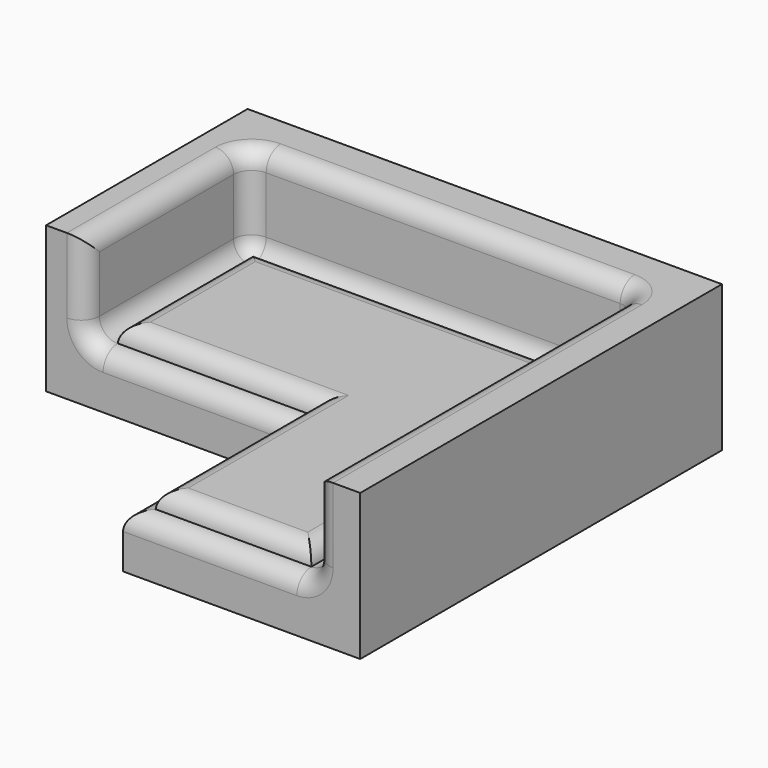
from build123d import *

# Parameters (mm, degrees)
F0_W          = 132.9678967595
F0_H          = 40.9901021048
F1_DEPTH      = 35.306
F2_W          = 109.3940883875
F2_H          = 52.1104875952
F3_DEPTH      = 57.15
F4_W          = 66.4839483798
F4_H          = 40.9901021048
F5_DEPTH      = 56.134
F6_W          = 53.8083352149
F6_H          = 26.0552437976
F7_DEPTH      = 59.69
F8_F1_R       = 5.08
F8_F2_R       = 5.08
F9_W          = 99.2340883875
F9_H          = 46.9125229284
F10_DEPTH     = 4.826
F11_W         = 43.6483352149
F11_H         = 56.2114770716
F12_DEPTH     = 4.826
F13_T1_DEPTH  = 56.3324502806
F13_T3_DEPTH  = 0.0774771487
F13_T5_DEPTH  = 68.8181149887
F13_T7_DEPTH  = 55.5857531726
F13_T9_DEPTH  = 115.8081150657
F13_T11_DEPTH = 99.2340883875
F13_T13_DEPTH = 59.5966379941
F13_T19_DEPTH = 68.2698682383
F13_T23_DEPTH = 12.7615922144


# Not quite as in the source:
# - a fillet or chamfer that OpenCascade refuses, or shapes differently, is made with other operations: its cross-section is extruded or revolved along the edge and cut away or added


with BuildPart() as f1:
    # F0 (on Front) → F1 (new body, symmetric)
    with BuildSketch(Plane.XZ):
        with Locations((0.8887089789, -5.8075287379)):
            Rectangle(F0_W, F0_H)
    extrude(amount=F1_DEPTH, both=True)

    # F2 (on face) → F3 (cut)
    with BuildSketch(Plane.XZ.offset(35.306)):
        with Locations((0, 14.6875223145)):
            Rectangle(F2_W, F2_H)
    extrude(amount=-F3_DEPTH, mode=Mode.SUBTRACT)

    # F4 (on face) → F5 (join)
    with BuildSketch(Plane.XZ.offset(35.306)):
        with Locations((34.1306831688, -5.8075287379)):
            Rectangle(F4_W, F4_H)
    extrude(amount=F5_DEPTH)

    # F6 (on face) → F7 (cut)
    with BuildSketch(Plane(origin=(0, -35.306, 0), x_dir=(-1, 0, 0), z_dir=(0, 1, 0))):
        with Locations((-27.7928765863, 1.6599004157)):
            Rectangle(F6_W, F6_H)
    extrude(amount=-F7_DEPTH, mode=Mode.SUBTRACT)

    # F8: fillet of radius 5.08 on 11 edges, made by hand

    # F8_f1
    f8_f1_edges = [f1.edges().sort_by_distance(p)[0] for p in [
        (-54.6970441937, -6.731, -11.3677214831),
        (-54.6970441937, 21.844, 1.6599004157),
        (0, 21.844, -11.3677214831),
        (54.6970441937, -34.798, -11.3677214831),
        (54.6970441937, 21.844, 1.6599004157),
    ]]
    fillet(f8_f1_edges, radius=F8_F1_R)

    # F8_f2
    f8_f2_edges = [f1.edges().sort_by_distance(p)[0] for p in [
        (-54.6970441937, -9.271, 14.6875223145),
        (0, 21.844, 14.6875223145),
        (54.6970441937, -37.338, 14.6875223145),
        (-24.3641676074, -35.306, -11.3677214831),
        (0.8887089789, -63.373, -11.3677214831),
        (25.2528765863, -91.44, -11.3677214831),
        (53.2091466422, -91.44, -9.8798239315),
        (-53.2091466422, -35.306, -9.8798239315),
        (53.2091466422, 20.3561024484, 14.6875223145),
        (-53.2091466422, 20.3561024484, 14.6875223145),
    ]]
    fillet(f8_f2_edges, radius=F8_F2_R)

    # F9 (on face) → F10 (join)
    with BuildSketch(Plane.XY.offset(-11.3677214831)):
        with Locations((0, -6.6922614642)):
            Rectangle(F9_W, F9_H)
    extrude(amount=F10_DEPTH)

    # F11 (on face) → F12 (join)
    with BuildSketch(Plane.XY.offset(-11.3677214831)):
        with Locations((27.7928765863, -58.2542614642)):
            Rectangle(F11_W, F11_H)
    extrude(amount=F12_DEPTH)

    # F13: fillet of radius 5.08 on 6 edges, made by hand

    # F13_s2 → F13_t1 (cut)
    with BuildSketch(Plane.YZ.offset(-6.7154060868)):
        with BuildLine():
            ThreePointArc((-81.2863539737, -6.5417214831), (-84.7875023567, -7.9409117896), (-86.36, -11.3677214831))
            Line((-86.36, -11.3677214831), (-86.36, -6.5417214831))
            Line((-86.36, -6.5417214831), (-81.2863539737, -6.5417214831))
        make_face()
    extrude(amount=F13_T1_DEPTH, mode=Mode.SUBTRACT)

    # F13_s4 → F13_t3 (cut)
    with BuildSketch(Plane.XZ.offset(30.1485229284)):
        with BuildLine():
            ThreePointArc((11.0423550052, -6.5417214831), (7.5412066221, -7.9409117896), (5.9687089789, -11.3677214831))
            Line((5.9687089789, -11.3677214831), (5.9687089789, -6.5417214831))
            Line((5.9687089789, -6.5417214831), (11.0423550052, -6.5417214831))
        make_face()
    extrude(amount=F13_T3_DEPTH, mode=Mode.SUBTRACT)

    # F13_s6 → F13_t5 (cut)
    with BuildSketch(Plane.XZ.offset(30.226000077)):
        with BuildLine():
            ThreePointArc((11.0423550052, -6.5417214831), (7.5412066221, -7.9409117896), (5.9687089789, -11.3677214831))
            Line((5.9687089789, -11.3677214831), (5.9687089789, -6.5417214831))
            Line((5.9687089789, -6.5417214831), (11.0423550052, -6.5417214831))
        make_face()
    extrude(amount=F13_T5_DEPTH, mode=Mode.SUBTRACT)

    # F13_s8 → F13_t7 (cut)
    with BuildSketch(Plane.YZ.offset(-49.6170441937)):
        with BuildLine():
            ThreePointArc((-25.0748769021, -6.5417214831), (-28.5760252851, -7.9409117896), (-30.1485229284, -11.3677214831))
            Line((-30.1485229284, -11.3677214831), (-30.1485229284, -6.5417214831))
            Line((-30.1485229284, -6.5417214831), (-25.0748769021, -6.5417214831))
        make_face()
    extrude(amount=F13_T7_DEPTH, mode=Mode.SUBTRACT)

    # F13_s10 → F13_t9 (cut)
    with BuildSketch(Plane.XZ.offset(-16.764)):
        with BuildLine():
            ThreePointArc((44.5433981675, -6.5417214831), (48.0445465505, -7.9409117896), (49.6170441937, -11.3677214831))
            Line((49.6170441937, -11.3677214831), (49.6170441937, -6.5417214831))
            Line((49.6170441937, -6.5417214831), (44.5433981675, -6.5417214831))
        make_face()
    extrude(amount=F13_T9_DEPTH, mode=Mode.SUBTRACT)

    # F13_s12 → F13_t11 (cut)
    with BuildSketch(Plane.YZ.offset(-49.6170441937)):
        with BuildLine():
            ThreePointArc((16.764, -11.3677214831), (15.1915023567, -7.9409117896), (11.6903539737, -6.5417214831))
            Line((11.6903539737, -6.5417214831), (16.764, -6.5417214831))
            Line((16.764, -6.5417214831), (16.764, -11.3677214831))
        make_face()
    extrude(amount=F13_T11_DEPTH, mode=Mode.SUBTRACT)

    # F13_s14 → F13_t13 (cut)
    with BuildSketch(Plane.XZ.offset(-16.764)):
        with BuildLine():
            ThreePointArc((-44.5433981675, -6.5417214831), (-48.0445465505, -7.9409117896), (-49.6170441937, -11.3677214831))
            Line((-49.6170441937, -11.3677214831), (-49.6170441937, -6.5417214831))
            Line((-49.6170441937, -6.5417214831), (-44.5433981675, -6.5417214831))
        make_face()
    extrude(amount=F13_T13_DEPTH, mode=Mode.SUBTRACT)


with BuildPart() as f13_tool17:
    # F13_s18 → F13_t19 (new body)
    with BuildSketch(Plane.YZ.offset(-49.6170441937)):
        with BuildLine():
            ThreePointArc((-25.0748769021, -6.5417214831), (-28.5760252851, -7.9409117896), (-30.1485229284, -11.3677214831))
            Line((-30.1485229284, -11.3677214831), (-30.1485229284, -6.5417214831))
            Line((-30.1485229284, -6.5417214831), (-25.0748769021, -6.5417214831))
        make_face()
    extrude(amount=F13_T19_DEPTH)

    split(bisect_by=Plane.YZ.offset(5.9687089789), keep=Keep.TOP)


with BuildPart() as f13_tool21:
    # F13_s22 → F13_t23 (new body)
    with BuildSketch(Plane.XZ.offset(17.4644078627)):
        with BuildLine():
            ThreePointArc((11.0423550052, -6.5417214831), (7.5412066221, -7.9409117896), (5.9687089789, -11.3677214831))
            Line((5.9687089789, -11.3677214831), (5.9687089789, -6.5417214831))
            Line((5.9687089789, -6.5417214831), (11.0423550052, -6.5417214831))
        make_face()
    extrude(amount=F13_T23_DEPTH)

    split(bisect_by=Plane.XZ.offset(30.1485229284), keep=Keep.BOTTOM)


with BuildPart() as f13_tool17_1:
    add(f13_tool17.part)

    # F13_t25: intersect F13_tool21
    add(f13_tool21.part, mode=Mode.INTERSECT)


with BuildPart() as f1_1:
    add(f1.part)

    # F13_t15: cut F13_tool17
    add(f13_tool17_1.part, mode=Mode.SUBTRACT)


solid = f1_1.part
